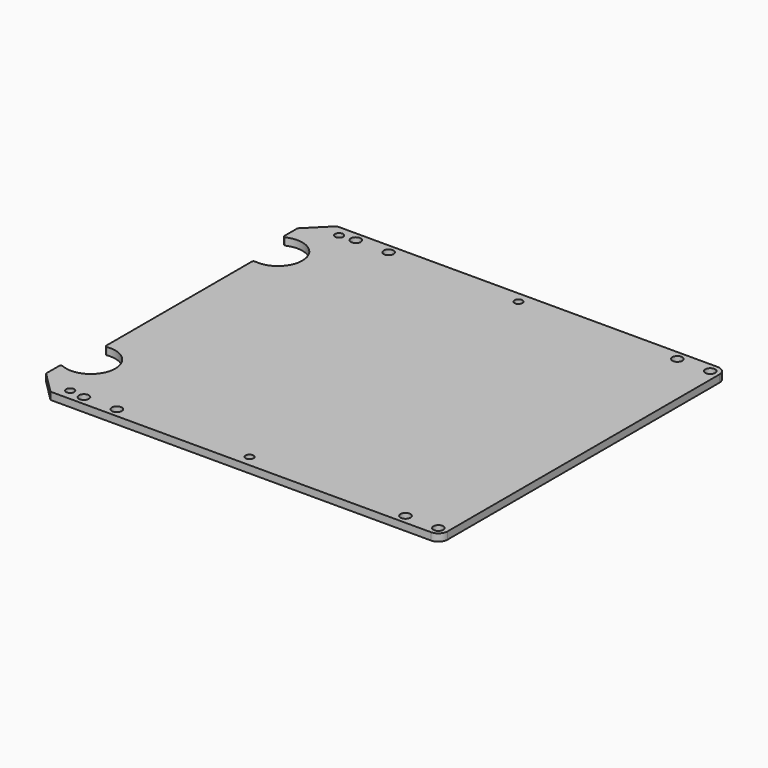
from build123d import *

# Parameters (mm, degrees)
F0_W     = 178.8466324
F0_H     = 155.575
F0_R     = 2.15265
F1_DEPTH = 3.175
F2_R     = 3.96875
F4_DEPTH = 3.175
F5_R     = 0.762
F6_SIZE  = 9.525
F7_R     = 1.7272
F8_DEPTH = 3.175


with BuildPart() as f1:
    # F0 (on Top) → F1 (new body)
    with BuildSketch(Plane.XY):
        with Locations((89.4233162, -77.7875)):
            Rectangle(F0_W, F0_H)
        with Locations((20.8903824, -151.60625)):
            Circle(F0_R, mode=Mode.SUBTRACT)
        with Locations((35.1778824, -151.60625)):
            Circle(F0_R, mode=Mode.SUBTRACT)
        with Locations((160.5903824, -151.60625)):
            Circle(F0_R, mode=Mode.SUBTRACT)
        with Locations((174.8778824, -151.60625)):
            Circle(F0_R, mode=Mode.SUBTRACT)
        with Locations((20.8903824, -3.96875)):
            Circle(F0_R, mode=Mode.SUBTRACT)
        with Locations((35.1778824, -3.96875)):
            Circle(F0_R, mode=Mode.SUBTRACT)
        with Locations((160.5903824, -3.96875)):
            Circle(F0_R, mode=Mode.SUBTRACT)
        with Locations((174.8778824, -3.96875)):
            Circle(F0_R, mode=Mode.SUBTRACT)
    extrude(amount=F1_DEPTH)

    # F2
    f2_edges = [f1.edges().sort_by_distance(p)[0] for p in [
        (178.846632, 0, 1.5875),
        (178.846632, -155.575, 1.5875),
    ]]
    fillet(f2_edges, radius=F2_R)

    # F3 (on face) → F4 (cut, through all)
    with BuildSketch(Plane.XY.offset(3.175)):
        with BuildLine():
            Line((0, -17.8102557702), (0, -137.7647442298))
            ThreePointArc((0, -137.7647442298), (15.9905975048, -130.293948325), (3.175, -118.1583617876))
            Line((3.175, -118.1583617876), (3.175, -37.4166382124))
            ThreePointArc((3.175, -37.4166382124), (15.9905975048, -25.281051675), (0, -17.8102557702))
        make_face()
    extrude(amount=-F4_DEPTH, mode=Mode.SUBTRACT)

    # F5
    f5_edges = [f1.edges().sort_by_distance(p)[0] for p in [
        (0, -17.810256, 1.5875),
        (0, -137.764744, 1.5875),
        (3.175, -37.416638, 1.5875),
        (3.175, -118.158362, 1.5875),
    ]]
    fillet(f5_edges, radius=F5_R)

    # F6
    f6_edges = [f1.edges().sort_by_distance(p)[0] for p in [
        (0, 0, 1.5875),
        (0, -155.575, 1.5875),
    ]]
    chamfer(f6_edges, length=F6_SIZE)

    # F7 (on face) → F8 (cut, through all)
    with BuildSketch(Plane.XY.offset(3.175)):
        with Locations((92.2014412, -4.7625)):
            Circle(F7_R)
        with Locations((14.2875, -4.7625)):
            Circle(F7_R)
        with Locations((14.2875, -150.8125)):
            Circle(F7_R)
        with Locations((92.2014412, -150.8125)):
            Circle(F7_R)
    extrude(amount=-F8_DEPTH, mode=Mode.SUBTRACT)


solid = f1.part
